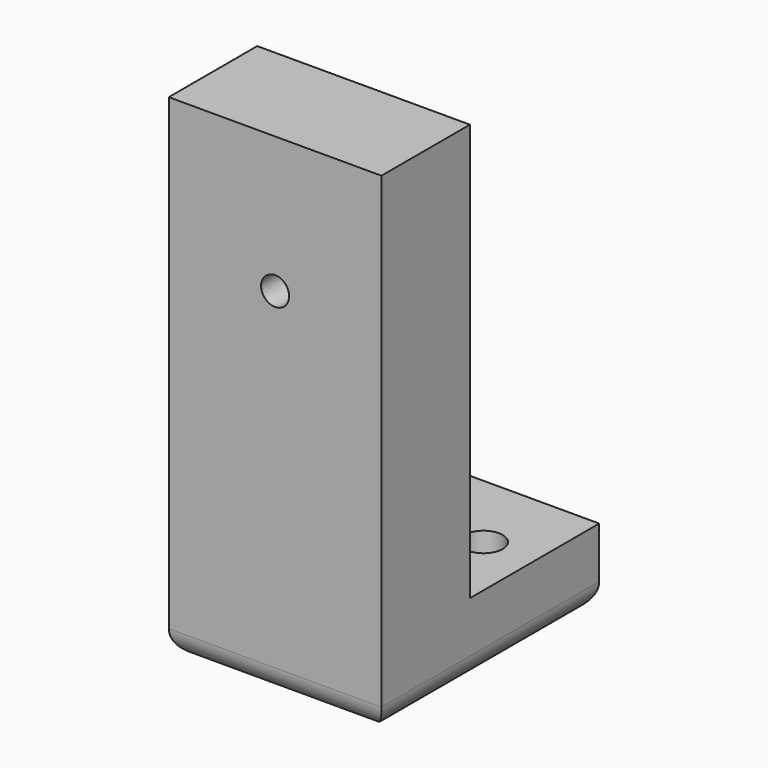
from build123d import *

# Parameters (mm, degrees)
F1_DEPTH       = 25
F3_D           = 4.4958
F3_CSINK_D     = 9.1186
F3_CSINK_ANGLE = 82
F5_D           = 3.3
F6_T1_DEPTH    = 40
F6_T3_DEPTH    = 47


# Not quite as in the source:
# - a fillet or chamfer that OpenCascade refuses, or shapes differently, is made with other operations: its cross-section is extruded or revolved along the edge and cut away or added


with BuildPart() as f1:
    # F0 (on Right) → F1 (new body)
    with BuildSketch(Plane.YZ):
        Polygon((-13, -58), (19, -58), (19, -49), (0, -49), (0, 0), (-13, 0), align=None)
    extrude(amount=F1_DEPTH)

    # F3 (through all)
    with Locations(Plane(origin=(0, 0, -58), x_dir=(1, 0, 0), z_dir=(0, 0, -1))):
        with Locations((6, -9.5), (19, -9.5)):
            CounterSinkHole(F3_D / 2, F3_CSINK_D / 2, counter_sink_angle=F3_CSINK_ANGLE)

    # F5 (through all)
    with Locations(Plane.XZ.offset(13)):
        with Locations((12.5, -16)):
            Hole(F5_D / 2)

    # F6: fillet of radius 3 on 4 edges, made by hand

    # F6_s2 → F6_t1 (cut)
    with BuildSketch(Plane.YZ.offset(-7.5)):
        with BuildLine():
            ThreePointArc((-10, -58), (-12.1213203436, -57.1213203436), (-13, -55))
            Line((-13, -55), (-13, -58))
            Line((-13, -58), (-10, -58))
        make_face()
        with BuildLine():
            ThreePointArc((16, -58), (18.1213203436, -57.1213203436), (19, -55))
            Line((19, -55), (19, -58))
            Line((19, -58), (16, -58))
        make_face()
    extrude(amount=F6_T1_DEPTH, mode=Mode.SUBTRACT)

    # F6_s4 → F6_t3 (cut)
    with BuildSketch(Plane.XZ.offset(-26.5)):
        with BuildLine():
            ThreePointArc((22, -58), (24.1213203436, -57.1213203436), (25, -55))
            Line((25, -55), (25, -58))
            Line((25, -58), (22, -58))
        make_face()
        with BuildLine():
            ThreePointArc((3, -58), (0.8786796564, -57.1213203436), (0, -55))
            Line((0, -55), (0, -58))
            Line((0, -58), (3, -58))
        make_face()
    extrude(amount=F6_T3_DEPTH, mode=Mode.SUBTRACT)


solid = f1.part
